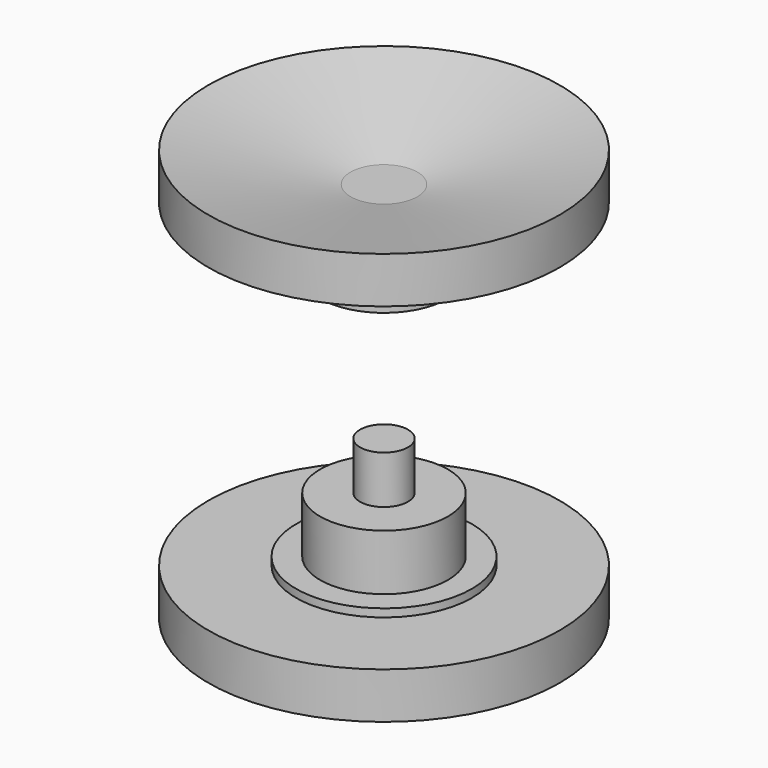
from build123d import *

# Parameters (mm, degrees)
F0_R     = 11
F0_R_2   = 5.5
F0_R_3   = 4
F0_R_4   = 1.5
F1_DEPTH = 1
F2_START = 1
F2_DEPTH = 0.5
F3_DEPTH = 5
F4_DEPTH = 8
F5_DEPTH = 2
F9_DEPTH = 6


# Not quite as in the source:
# - a fillet or chamfer that OpenCascade refuses, or shapes differently, is made with other operations: its cross-section is extruded or revolved along the edge and cut away or added


with BuildPart() as f1:
    # F0 (on Top) → F1 (new body)
    with BuildSketch(Plane.XY):
        Circle(F0_R)
        Circle(F0_R_2, mode=Mode.SUBTRACT)
        Circle(F0_R_2)
        Circle(F0_R_3, mode=Mode.SUBTRACT)
        Circle(F0_R_3)
        Circle(F0_R_4, mode=Mode.SUBTRACT)
        Circle(F0_R_4)
    extrude(amount=F1_DEPTH)

    # F0 (on Top) → F2 (join)
    with BuildSketch(Plane.XY.offset(F2_START)):
        Circle(F0_R_2)
        Circle(F0_R_3, mode=Mode.SUBTRACT)
    extrude(amount=F2_DEPTH)

    # F0 (on Top) → F3 (join)
    with BuildSketch(Plane.XY):
        Circle(F0_R_3)
        Circle(F0_R_4, mode=Mode.SUBTRACT)
    extrude(amount=F3_DEPTH)

    # F0 (on Top) → F4 (join)
    with BuildSketch(Plane.XY):
        Circle(F0_R_4)
    extrude(amount=F4_DEPTH)

    # F0 (on Top) → F5 (join)
    with BuildSketch(Plane.XY):
        Circle(F0_R)
        Circle(F0_R_2, mode=Mode.SUBTRACT)
        Circle(F0_R_2)
        Circle(F0_R_3, mode=Mode.SUBTRACT)
        Circle(F0_R_3)
        Circle(F0_R_4, mode=Mode.SUBTRACT)
    extrude(amount=-F5_DEPTH)

    # F6: chamfer of 10 x 2.1255656167 on 1 edges, made by hand


with BuildPart() as f6_tool2:
    # F6_s3 → F6_t4 (revolve)
    with BuildSketch(Plane.XZ):
        Polygon((11.5, -2), (1.5, 0.1255656167), (1.5, -2), align=None)
    revolve(axis=Axis((0, 0, -2), (0, 0, 1)))

    split(bisect_by=Plane.XY, keep=Keep.BOTTOM)


with BuildPart() as f1_1:
    add(f1.part)

    # F6_t1: cut F6_tool2
    add(f6_tool2.part, mode=Mode.SUBTRACT)


with BuildPart() as f8_1:
    # F8: instance of F1
    add(f1_1.part.mirror(Plane.XY.offset(11)))

    # F9 (cut): a face of the model
    f9_faces = [f8_1.faces().sort_by_distance(p)[0] for p in [
        (0, 0, 14),
    ]]
    extrude(f9_faces, amount=-F9_DEPTH, mode=Mode.SUBTRACT)


solid = Compound([f1_1.part, f8_1.part])
